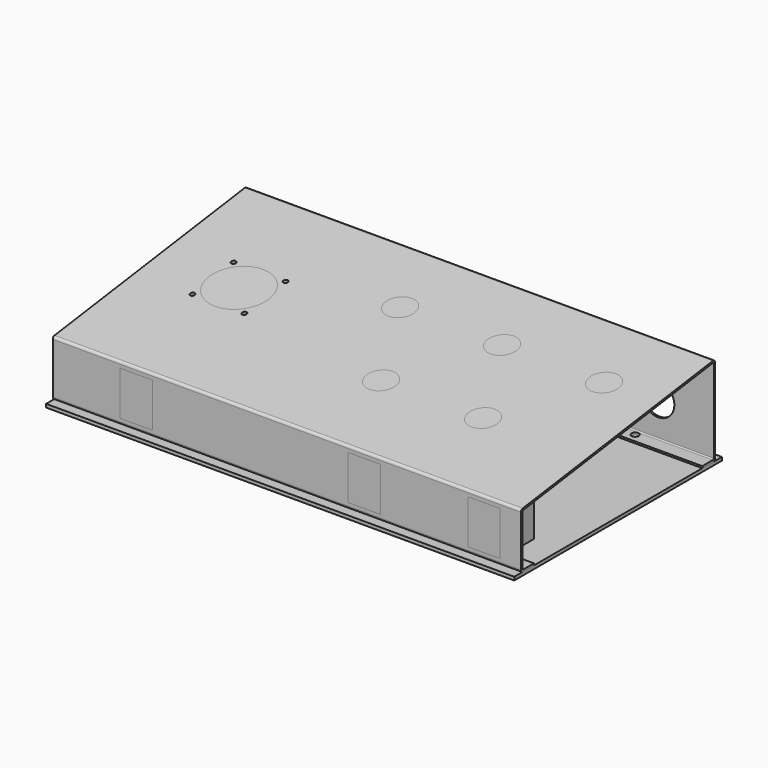
from build123d import *

# Parameters (mm, degrees)
F3_W      = 320.675
F3_H      = 167.9854784825
F3_R      = 1.5875
F3_R_2    = 20.6375
F9_DEPTH  = 1.27
F0_W      = 320.675
F0_H      = 38.1
F0_W_2    = 22.0218
F0_H_2    = 30.226
F10_DEPTH = 1.27
F7_W      = 320.675
F7_H      = 61.341
F7_R      = 11.1125
F11_DEPTH = 1.27
F13_DEPTH = 320.676
F8_W      = 320.675
F8_H      = 11.1125
F8_R      = 2.5019
F14_DEPTH = 1.27
F15_R     = 1.778
F16_R     = 0.762
F17_DEPTH = 25.4254
F18_DEPTH = 8.382
F19_DEPTH = 26.27
F20_W     = 320.675
F20_H     = 9.3345
F20_R     = 2.5019
F20_H_2   = 7.493
F21_DEPTH = 2.286
F22_DEPTH = 1.27
F23_DEPTH = 22.6822
F24_DEPTH = 29.0068


with BuildPart() as f9:
    # F3 (on face) → F9 (new body)
    with BuildSketch(Plane(origin=(0, -5.2204906409, 37.3707253532), x_dir=(1, 0, 0), z_dir=(0, -0.1383512445, 0.9903832254))):
        with Locations((160.3375, 89.2639216554)):
            Rectangle(F3_W, F3_H)
        with BuildLine():
            Line((39.37, 118.3011824141), (74.93, 118.3011824141))
            ThreePointArc((74.93, 118.3011824141), (79.4201280605, 116.4413104746), (81.28, 111.9511824141))
            Line((81.28, 111.9511824141), (81.28, 76.3911824141))
            ThreePointArc((81.28, 76.3911824141), (79.4201280605, 71.9010543536), (74.93, 70.0411824141))
            Line((74.93, 70.0411824141), (39.37, 70.0411824141))
            ThreePointArc((39.37, 70.0411824141), (34.8798719395, 71.9010543536), (33.02, 76.3911824141))
            Line((33.02, 76.3911824141), (33.02, 111.9511824141))
            ThreePointArc((33.02, 111.9511824141), (34.8798719395, 116.4413104746), (39.37, 118.3011824141))
        make_face(mode=Mode.SUBTRACT)
        with BuildLine():
            ThreePointArc((203.36, 124.4171196413), (213.36, 134.4171196413), (223.36, 124.4171196413))
            Line((223.36, 124.4171196413), (273.21, 124.4171196413))
            ThreePointArc((273.21, 124.4171196413), (283.21, 134.4171196413), (293.21, 124.4171196413))
            ThreePointArc((293.21, 124.4171196413), (288.21, 115.7568656034), (278.21, 115.7568656034))
            Line((278.21, 115.7568656034), (253.285, 72.5854992248))
            ThreePointArc((253.285, 72.5854992248), (256.9452540378, 68.9252451869), (258.285, 63.9252451869))
            ThreePointArc((258.285, 63.9252451869), (248.285, 53.9252451869), (238.285, 63.9252451869))
            Line((238.285, 63.9252451869), (213.36, 63.9252451869))
            Line((213.36, 63.9252451869), (188.435, 63.9252451869))
            ThreePointArc((188.435, 63.9252451869), (173.435, 55.2649911491), (173.435, 72.5854992248))
            Line((173.435, 72.5854992248), (148.51, 115.7568656034))
            ThreePointArc((148.51, 115.7568656034), (134.8497459622, 129.4171196413), (153.51, 124.4171196413))
            Line((153.51, 124.4171196413), (203.36, 124.4171196413))
        make_face(mode=Mode.SUBTRACT)
        with BuildLine():
            ThreePointArc((208.36, 115.7568656034), (204.6997459622, 119.4171196413), (203.36, 124.4171196413))
            Line((203.36, 124.4171196413), (153.51, 124.4171196413))
            ThreePointArc((153.51, 124.4171196413), (152.1702540378, 119.4171196413), (148.51, 115.7568656034))
            Line((148.51, 115.7568656034), (173.435, 72.5854992248))
            ThreePointArc((173.435, 72.5854992248), (178.435, 73.9252451869), (183.435, 72.5854992248))
            Line((183.435, 72.5854992248), (208.36, 115.7568656034))
        make_face()
        with BuildLine():
            ThreePointArc((213.36, 114.4171196413), (210.771809549, 114.7578613784), (208.36, 115.7568656034))
            Line((208.36, 115.7568656034), (183.435, 72.5854992248))
            ThreePointArc((183.435, 72.5854992248), (187.0952540378, 68.9252451869), (188.435, 63.9252451869))
            Line((188.435, 63.9252451869), (213.36, 63.9252451869))
            Line((213.36, 63.9252451869), (213.36, 114.4171196413))
        make_face()
        with BuildLine():
            Line((243.285, 72.5854992248), (218.36, 115.7568656034))
            ThreePointArc((218.36, 115.7568656034), (215.948190451, 114.7578613784), (213.36, 114.4171196413))
            Line((213.36, 114.4171196413), (213.36, 63.9252451869))
            Line((213.36, 63.9252451869), (238.285, 63.9252451869))
            ThreePointArc((238.285, 63.9252451869), (239.6247459622, 68.9252451869), (243.285, 72.5854992248))
        make_face()
        with BuildLine():
            Line((273.21, 124.4171196413), (223.36, 124.4171196413))
            ThreePointArc((223.36, 124.4171196413), (222.0202540378, 119.4171196413), (218.36, 115.7568656034))
            Line((218.36, 115.7568656034), (243.285, 72.5854992248))
            ThreePointArc((243.285, 72.5854992248), (248.285, 73.9252451869), (253.285, 72.5854992248))
            Line((253.285, 72.5854992248), (278.21, 115.7568656034))
            ThreePointArc((278.21, 115.7568656034), (274.5497459622, 119.4171196413), (273.21, 124.4171196413))
        make_face()
        with BuildLine():
            ThreePointArc((81.28, 111.9511824141), (79.4201280605, 116.4413104746), (74.93, 118.3011824141))
            Line((74.93, 118.3011824141), (39.37, 118.3011824141))
            ThreePointArc((39.37, 118.3011824141), (34.8798719395, 116.4413104746), (33.02, 111.9511824141))
            Line((33.02, 111.9511824141), (33.02, 76.3911824141))
            ThreePointArc((33.02, 76.3911824141), (34.8798719395, 71.9010543536), (39.37, 70.0411824141))
            Line((39.37, 70.0411824141), (74.93, 70.0411824141))
            ThreePointArc((74.93, 70.0411824141), (79.4201280605, 71.9010543536), (81.28, 76.3911824141))
            Line((81.28, 76.3911824141), (81.28, 111.9511824141))
        make_face()
        with Locations((39.37, 76.3911824141)):
            Circle(F3_R, mode=Mode.SUBTRACT)
        with Locations((74.93, 76.3911824141)):
            Circle(F3_R, mode=Mode.SUBTRACT)
        with Locations((57.15, 94.1711824141)):
            Circle(F3_R_2, mode=Mode.SUBTRACT)
        with Locations((39.37, 111.9511824141)):
            Circle(F3_R, mode=Mode.SUBTRACT)
        with Locations((74.93, 111.9511824141)):
            Circle(F3_R, mode=Mode.SUBTRACT)
    extrude(amount=-F9_DEPTH)

    # F0 (on Front) → F10 (join)
    with BuildSketch(Plane.XZ):
        with Locations((160.3375, 19.05)):
            Rectangle(F0_W, F0_H)
        with Locations((57.15, 19.05)):
            Rectangle(F0_W_2, F0_H_2, mode=Mode.SUBTRACT)
        with Locations((213.36, 19.05)):
            Rectangle(F0_W_2, F0_H_2, mode=Mode.SUBTRACT)
        with Locations((295.275, 19.05)):
            Rectangle(F0_W_2, F0_H_2, mode=Mode.SUBTRACT)
    extrude(amount=-F10_DEPTH)

    # F7 (on face) → F11 (join)
    with BuildSketch(Plane(origin=(0, 166.37, 0), x_dir=(-1, 0, 0), z_dir=(0, 1, 0))):
        with Locations((-160.3375, 30.6705)):
            Rectangle(F7_W, F7_H)
        with Locations((-282.575, 25.4)):
            Circle(F7_R, mode=Mode.SUBTRACT)
        with Locations((-38.1, 25.4)):
            Circle(F7_R, mode=Mode.SUBTRACT)
    extrude(amount=-F11_DEPTH)

    # F12 (on face) → F13 (cut, through all)
    with BuildSketch(Plane(origin=(320.675, 0, 0), x_dir=(0, -1, 0), z_dir=(-1, 0, 0))):
        Polygon((-165.1, 61.1635877863), (-165.1, 61.341), (-166.37, 61.341), align=None)
        Polygon((-166.37, 60.0586681032), (-166.37, 61.341), (-166.5457060805, 60.0832133037), align=None)
    extrude(amount=F13_DEPTH, mode=Mode.SUBTRACT)

    # F8 (on Top) → F14 (join)
    with BuildSketch(Plane.XY):
        with Locations((160.3375, 5.55625)):
            Rectangle(F8_W, F8_H)
        with Locations((50.8, 5.08)):
            Circle(F8_R, mode=Mode.SUBTRACT)
        with Locations((269.875, 5.08)):
            Circle(F8_R, mode=Mode.SUBTRACT)
        with Locations((160.3375, 160.81375)):
            Rectangle(F8_W, F8_H)
        with Locations((50.8, 161.29)):
            Circle(F8_R, mode=Mode.SUBTRACT)
        with Locations((269.875, 161.29)):
            Circle(F8_R, mode=Mode.SUBTRACT)
    extrude(amount=F14_DEPTH)

    # F15
    f15_edges = [f9.edges().sort_by_distance(p)[0] for p in [
        (160.3375, 0, 38.1),
        (160.3375, 166.37, 61.341),
        (160.3375, 166.37, 0),
        (160.3375, 0, 0),
    ]]
    fillet(f15_edges, radius=F15_R)

    # F16
    f16_edges = [f9.edges().sort_by_distance(p)[0] for p in [
        (160.3375, 165.1, 59.881256),
        (160.3375, 1.27, 36.99508),
        (160.3375, 1.27, 1.27),
        (160.3375, 165.1, 1.27),
    ]]
    fillet(f16_edges, radius=F16_R)


with BuildPart() as f17:
    # F3 (on face) → F17 (new body)
    with BuildSketch(Plane(origin=(0, -5.2204906409, 37.3707253532), x_dir=(1, 0, 0), z_dir=(0, -0.1383512445, 0.9903832254))):
        with Locations((57.15, 94.1711824141)):
            Circle(F3_R_2)
    extrude(amount=-F17_DEPTH)

    # F3 (on face) → F18 (join)
    with BuildSketch(Plane(origin=(0, -5.2204906409, 37.3707253532), x_dir=(1, 0, 0), z_dir=(0, -0.1383512445, 0.9903832254))):
        with BuildLine():
            ThreePointArc((81.28, 111.9511824141), (79.4201280605, 116.4413104746), (74.93, 118.3011824141))
            Line((74.93, 118.3011824141), (39.37, 118.3011824141))
            ThreePointArc((39.37, 118.3011824141), (34.8798719395, 116.4413104746), (33.02, 111.9511824141))
            Line((33.02, 111.9511824141), (33.02, 76.3911824141))
            ThreePointArc((33.02, 76.3911824141), (34.8798719395, 71.9010543536), (39.37, 70.0411824141))
            Line((39.37, 70.0411824141), (74.93, 70.0411824141))
            ThreePointArc((74.93, 70.0411824141), (79.4201280605, 71.9010543536), (81.28, 76.3911824141))
            Line((81.28, 76.3911824141), (81.28, 111.9511824141))
        make_face()
        with Locations((39.37, 76.3911824141)):
            Circle(F3_R, mode=Mode.SUBTRACT)
        with Locations((74.93, 76.3911824141)):
            Circle(F3_R, mode=Mode.SUBTRACT)
        with Locations((57.15, 94.1711824141)):
            Circle(F3_R_2, mode=Mode.SUBTRACT)
        with Locations((39.37, 111.9511824141)):
            Circle(F3_R, mode=Mode.SUBTRACT)
        with Locations((74.93, 111.9511824141)):
            Circle(F3_R, mode=Mode.SUBTRACT)
    extrude(amount=-F18_DEPTH)

    # F3 (on face) → F22 (cut, through all)
    with BuildSketch(Plane(origin=(0, -5.2204906409, 37.3707253532), x_dir=(1, 0, 0), z_dir=(0, -0.1383512445, 0.9903832254))):
        with BuildLine():
            ThreePointArc((81.28, 111.9511824141), (79.4201280605, 116.4413104746), (74.93, 118.3011824141))
            Line((74.93, 118.3011824141), (39.37, 118.3011824141))
            ThreePointArc((39.37, 118.3011824141), (34.8798719395, 116.4413104746), (33.02, 111.9511824141))
            Line((33.02, 111.9511824141), (33.02, 76.3911824141))
            ThreePointArc((33.02, 76.3911824141), (34.8798719395, 71.9010543536), (39.37, 70.0411824141))
            Line((39.37, 70.0411824141), (74.93, 70.0411824141))
            ThreePointArc((74.93, 70.0411824141), (79.4201280605, 71.9010543536), (81.28, 76.3911824141))
            Line((81.28, 76.3911824141), (81.28, 111.9511824141))
        make_face()
        with Locations((39.37, 76.3911824141)):
            Circle(F3_R, mode=Mode.SUBTRACT)
        with Locations((74.93, 76.3911824141)):
            Circle(F3_R, mode=Mode.SUBTRACT)
        with Locations((57.15, 94.1711824141)):
            Circle(F3_R_2, mode=Mode.SUBTRACT)
        with Locations((39.37, 111.9511824141)):
            Circle(F3_R, mode=Mode.SUBTRACT)
        with Locations((74.93, 111.9511824141)):
            Circle(F3_R, mode=Mode.SUBTRACT)
    extrude(amount=-F22_DEPTH, mode=Mode.SUBTRACT)


with BuildPart() as f19:
    # F3 (on face) → F19 (new body)
    with BuildSketch(Plane(origin=(0, -5.2204906409, 37.3707253532), x_dir=(1, 0, 0), z_dir=(0, -0.1383512445, 0.9903832254))):
        with BuildLine():
            ThreePointArc((293.21, 124.4171196413), (283.21, 134.4171196413), (273.21, 124.4171196413))
            Line((273.21, 124.4171196413), (283.21, 124.4171196413))
            Line((283.21, 124.4171196413), (278.21, 115.7568656034))
            ThreePointArc((278.21, 115.7568656034), (288.21, 115.7568656034), (293.21, 124.4171196413))
        make_face()
        with BuildLine():
            Line((283.21, 124.4171196413), (273.21, 124.4171196413))
            ThreePointArc((273.21, 124.4171196413), (274.5497459622, 119.4171196413), (278.21, 115.7568656034))
            Line((278.21, 115.7568656034), (283.21, 124.4171196413))
        make_face()
    extrude(amount=-F19_DEPTH)


with BuildPart() as f19b:
    # F3 (on face) → F19, piece 2 (new body)
    with BuildSketch(Plane(origin=(0, -5.2204906409, 37.3707253532), x_dir=(1, 0, 0), z_dir=(0, -0.1383512445, 0.9903832254))):
        with BuildLine():
            ThreePointArc((218.36, 115.7568656034), (222.0202540378, 119.4171196413), (223.36, 124.4171196413))
            Line((223.36, 124.4171196413), (213.36, 124.4171196413))
            Line((213.36, 124.4171196413), (218.36, 115.7568656034))
        make_face()
        with BuildLine():
            ThreePointArc((213.36, 114.4171196413), (215.948190451, 114.7578613784), (218.36, 115.7568656034))
            Line((218.36, 115.7568656034), (213.36, 124.4171196413))
            Line((213.36, 124.4171196413), (213.36, 114.4171196413))
        make_face()
        with BuildLine():
            Line((213.36, 114.4171196413), (213.36, 124.4171196413))
            Line((213.36, 124.4171196413), (208.36, 115.7568656034))
            ThreePointArc((208.36, 115.7568656034), (210.771809549, 114.7578613784), (213.36, 114.4171196413))
        make_face()
        with BuildLine():
            Line((213.36, 124.4171196413), (203.36, 124.4171196413))
            ThreePointArc((203.36, 124.4171196413), (204.6997459622, 119.4171196413), (208.36, 115.7568656034))
            Line((208.36, 115.7568656034), (213.36, 124.4171196413))
        make_face()
        with BuildLine():
            Line((213.36, 124.4171196413), (223.36, 124.4171196413))
            ThreePointArc((223.36, 124.4171196413), (213.36, 134.4171196413), (203.36, 124.4171196413))
            Line((203.36, 124.4171196413), (213.36, 124.4171196413))
        make_face()
    extrude(amount=-F19_DEPTH)


with BuildPart() as f19c:
    # F3 (on face) → F19, piece 3 (new body)
    with BuildSketch(Plane(origin=(0, -5.2204906409, 37.3707253532), x_dir=(1, 0, 0), z_dir=(0, -0.1383512445, 0.9903832254))):
        with BuildLine():
            Line((143.51, 124.4171196413), (153.51, 124.4171196413))
            ThreePointArc((153.51, 124.4171196413), (134.8497459622, 129.4171196413), (148.51, 115.7568656034))
            Line((148.51, 115.7568656034), (143.51, 124.4171196413))
        make_face()
        with BuildLine():
            ThreePointArc((148.51, 115.7568656034), (152.1702540378, 119.4171196413), (153.51, 124.4171196413))
            Line((153.51, 124.4171196413), (143.51, 124.4171196413))
            Line((143.51, 124.4171196413), (148.51, 115.7568656034))
        make_face()
    extrude(amount=-F19_DEPTH)


with BuildPart() as f19d:
    # F3 (on face) → F19, piece 4 (new body)
    with BuildSketch(Plane(origin=(0, -5.2204906409, 37.3707253532), x_dir=(1, 0, 0), z_dir=(0, -0.1383512445, 0.9903832254))):
        with BuildLine():
            Line((178.435, 63.9252451869), (183.435, 72.5854992248))
            ThreePointArc((183.435, 72.5854992248), (178.435, 73.9252451869), (173.435, 72.5854992248))
            Line((173.435, 72.5854992248), (178.435, 63.9252451869))
        make_face()
        with BuildLine():
            ThreePointArc((188.435, 63.9252451869), (187.0952540378, 68.9252451869), (183.435, 72.5854992248))
            Line((183.435, 72.5854992248), (178.435, 63.9252451869))
            Line((178.435, 63.9252451869), (188.435, 63.9252451869))
        make_face()
        with BuildLine():
            ThreePointArc((173.435, 72.5854992248), (173.435, 55.2649911491), (188.435, 63.9252451869))
            Line((188.435, 63.9252451869), (178.435, 63.9252451869))
            Line((178.435, 63.9252451869), (173.435, 72.5854992248))
        make_face()
    extrude(amount=-F19_DEPTH)


with BuildPart() as f19e:
    # F3 (on face) → F19, piece 5 (new body)
    with BuildSketch(Plane(origin=(0, -5.2204906409, 37.3707253532), x_dir=(1, 0, 0), z_dir=(0, -0.1383512445, 0.9903832254))):
        with BuildLine():
            ThreePointArc((253.285, 72.5854992248), (248.285, 73.9252451869), (243.285, 72.5854992248))
            Line((243.285, 72.5854992248), (248.285, 63.9252451869))
            Line((248.285, 63.9252451869), (253.285, 72.5854992248))
        make_face()
        with BuildLine():
            Line((248.285, 63.9252451869), (243.285, 72.5854992248))
            ThreePointArc((243.285, 72.5854992248), (239.6247459622, 68.9252451869), (238.285, 63.9252451869))
            Line((238.285, 63.9252451869), (248.285, 63.9252451869))
        make_face()
        with BuildLine():
            ThreePointArc((258.285, 63.9252451869), (256.9452540378, 68.9252451869), (253.285, 72.5854992248))
            Line((253.285, 72.5854992248), (248.285, 63.9252451869))
            Line((248.285, 63.9252451869), (238.285, 63.9252451869))
            ThreePointArc((238.285, 63.9252451869), (248.285, 53.9252451869), (258.285, 63.9252451869))
        make_face()
    extrude(amount=-F19_DEPTH)


with BuildPart() as f21:
    # F20 (on face) → F21 (new body)
    with BuildSketch(Plane(origin=(0, 0, 0), x_dir=(1, 0, 0), z_dir=(0, 0, -1))):
        with Locations((160.3375, -159.92475)):
            Rectangle(F20_W, F20_H)
        with Locations((50.8, -161.29)):
            Circle(F20_R, mode=Mode.SUBTRACT)
        with Locations((269.875, -161.29)):
            Circle(F20_R, mode=Mode.SUBTRACT)
        Polygon((0, -11.1125), (0, -155.2575), (320.675, -155.2575), (320.675, -11.1125), (320.675, -1.778), (320.675, 5.715), (0, 5.715), (0, -1.778), align=None)
        with Locations((50.8, -5.08)):
            Circle(F20_R, mode=Mode.SUBTRACT)
        with Locations((269.875, -5.08)):
            Circle(F20_R, mode=Mode.SUBTRACT)
        with Locations((160.3375, -168.3385)):
            Rectangle(F20_W, F20_H_2)
    extrude(amount=F21_DEPTH)


with BuildPart() as f23:
    # F0 (on Front) → F23 (new body)
    with BuildSketch(Plane.XZ):
        with Locations((57.15, 19.05)):
            Rectangle(F0_W_2, F0_H_2)
    extrude(amount=-F23_DEPTH)


with BuildPart() as f23b:
    # F0 (on Front) → F23, piece 2 (new body)
    with BuildSketch(Plane.XZ):
        with Locations((213.36, 19.05)):
            Rectangle(F0_W_2, F0_H_2)
    extrude(amount=-F23_DEPTH)


with BuildPart() as f24:
    # F0 (on Front) → F24 (new body)
    with BuildSketch(Plane.XZ):
        with Locations((295.275, 19.05)):
            Rectangle(F0_W_2, F0_H_2)
    extrude(amount=-F24_DEPTH)


solid = Compound([f9.part, f17.part, f19.part, f19b.part, f19c.part, f19d.part, f19e.part, f21.part, f23.part, f23b.part, f24.part])
